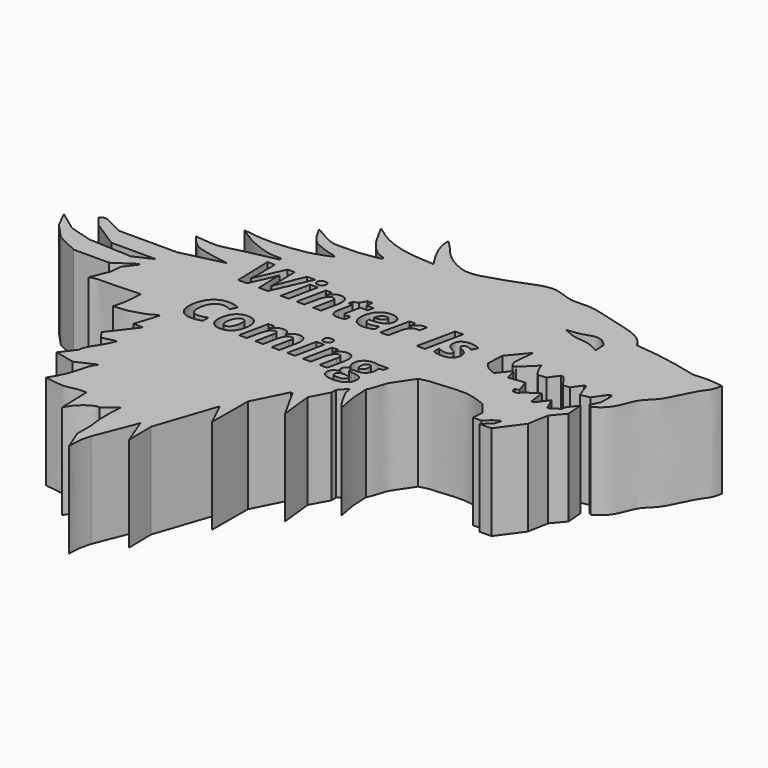
from build123d import *

# Parameters (mm, degrees)
F1_DEPTH     = 25
F2_R         = 94.3461279021
F3_DEPTH     = 25
F5_TEXT_SIZE = 14.0094855892
F6_DEPTH     = 25


# Not quite as in the source:
# - Text() gives the source's letters only with a copy of the font that has no kerning and outlines rounded to 1/6400 em; it was checked with that copy


with BuildPart() as f1:
    # F0 (on Top) → F1 (new body)
    with BuildSketch(Plane.XY):
        with BuildLine():
            add(Edge.make_bspline(
                [(8.3714025095, 46.0173152387), (11.1521832152, 46.754596787), (16.3296971789, 48.4982359497), (24.1106627679, 52.0612451404), (29.6085529308, 48.7695111991), (35.133174344, 49.9703703897), (43.252929809, 46.964556813), (51.3283334626, 45.612910231), (52.9993437231, 42.0622937381)],
                knots=[0, 0, 0, 0, 0.1755033114, 0.3449978942, 0.4876629093, 0.6241423562, 0.8019542951, 1, 1, 1, 1], degree=3))
            add(Edge.make_bspline(
                [(-6.1449650675, 54.0423952043), (-5.6293203869, 53.5672210533), (-4.3756327313, 52.4119294547), (-1.6804544816, 48.6615797252), (4.3028583968, 45.283770124), (7.1379722318, 45.7949318186), (8.3714025095, 46.0173152387)],
                knots=[0, 0, 0, 0, 0.18314369, 0.4452775175, 0.758665244, 1, 1, 1, 1], degree=3))
            add(Edge.make_bspline(
                [(-2.1649692208, 44.1456995904), (-2.6830426714, 44.902201383), (-3.8678058954, 46.6322176608), (-6.1266059516, 51.2050741718), (-6.1394772709, 53.1942802552), (-6.1449650675, 54.0423952043)],
                knots=[0, 0, 0, 0, 0.3083257044, 0.7050987754, 1, 1, 1, 1], degree=3))
            add(Edge.make_bspline(
                [(-20.5234307796, 49.826964736), (-19.2660471951, 48.8893211458), (-16.5760607157, 46.8833711627), (-10.5835555234, 44.6421995592), (-5.1143142903, 44.3196420651), (-2.1649692208, 44.1456995904)],
                knots=[0, 0, 0, 0, 0.2879457207, 0.6160173435, 1, 1, 1, 1], degree=3))
            add(Edge.make_bspline(
                [(-11.792646721, 39.9065613747), (-12.7415984122, 40.1991817878), (-14.864454764, 40.8537895075), (-17.9140349598, 44.889493557), (-18.9338887823, 46.9178849726), (-19.9665200349, 48.807741727), (-20.5234307796, 49.826964736)],
                knots=[0, 0, 0, 0, 0.242668036, 0.5428615453, 0.7534596047, 1, 1, 1, 1], degree=3))
            Line((-11.792646721, 39.9065613747), (-12.1578518301, 39.2757542431))
            Line((-12.1578518301, 39.2757542431), (-17.669133842, 38.4789407253))
            add(Edge.make_bspline(
                [(-30.1525183022, 41.5333881974), (-29.4462955799, 41.1485654195), (-27.8722301429, 40.2908526681), (-24.4388988209, 38.1832992198), (-20.9659487244, 38.4500592903), (-18.7606144745, 38.4693789125), (-17.669133842, 38.4789407253)],
                knots=[0, 0, 0, 0, 0.2218830142, 0.4945442459, 0.7498360323, 1, 1, 1, 1], degree=3))
            add(Edge.make_bspline(
                [(-20.9172498435, 34.4844385982), (-22.0652264332, 34.5773157469), (-24.8199894343, 35.715890512), (-27.6018886219, 36.794447921), (-29.4810709407, 40.069825786), (-30.1525183022, 41.5333881974)],
                knots=[0, 0, 0, 0, 0.3311370823, 0.6221258171, 1, 1, 1, 1], degree=3))
            add(Edge.make_bspline(
                [(-20.7182727754, 33.6885266006), (-20.3961660871, 33.7569314037), (-20.0173134256, 34.0869757025), (-20.4925501201, 34.2820213144), (-20.9172498435, 34.4844385982)],
                knots=[0, 0, 0, 0, 0.4600614089, 1, 1, 1, 1], degree=3))
            add(Edge.make_bspline(
                [(-41.9234707952, 31.6619388759), (-40.2252279309, 31.4070143382), (-36.7717771519, 30.8886141953), (-31.412260856, 31.079758672), (-24.6846617301, 32.0754797978), (-21.932813416, 33.1945985165), (-20.7182727754, 33.6885266006)],
                knots=[0, 0, 0, 0, 0.2445734873, 0.4973508312, 0.7781535267, 1, 1, 1, 1], degree=3))
            add(Edge.make_bspline(
                [(-28.4772720188, 26.5822634101), (-29.4158292377, 26.5659337389), (-31.6836604975, 26.5264764335), (-37.6292895418, 28.7001284099), (-40.5298935718, 30.7007517807), (-41.9234707952, 31.6619388759)],
                knots=[0, 0, 0, 0, 0.2683864124, 0.6485007876, 1, 1, 1, 1], degree=3))
            ThreePointArc((-28.4772720188, 26.5822634101), (-28.1204352447, 26.2336581945), (-28.4772720188, 25.885052979))
            add(Edge.make_bspline(
                [(-47.9933172464, 23.3067888767), (-45.9689231613, 23.0397900521), (-42.1158191567, 22.5316013316), (-37.515328371, 24.0476780795), (-31.8113888815, 25.2072498766), (-28.4772720188, 25.885052979)],
                knots=[0, 0, 0, 0, 0.3150353706, 0.5996184522, 1, 1, 1, 1], degree=3))
            add(Edge.make_bspline(
                [(-35.507440567, 17.9841239005), (-37.7337411291, 18.2148626084), (-41.7881476434, 19.1150723529), (-45.0286914617, 19.7872195383), (-47.2463314192, 22.1207634071), (-47.9933172464, 23.3067888767)],
                knots=[0, 0, 0, 0, 0.3933673205, 0.675332231, 1, 1, 1, 1], degree=3))
            add(Edge.make_bspline(
                [(-46.6502159834, 15.3476633132), (-44.9365327779, 15.7569410645), (-41.3990675416, 16.601791392), (-37.5116464679, 17.5138838493), (-35.507440567, 17.9841239005)],
                knots=[0, 0, 0, 0, 0.4844381756, 1, 1, 1, 1], degree=3))
            Line((-46.6502159834, 15.3476633132), (-62.0212741196, 15.3476633132))
            Line((-62.0212741196, 15.3476633132), (-66.7967498302, 17.8348906338))
            add(Edge.make_bspline(
                [(-68.9357668161, 17.4369327724), (-68.6066134375, 17.6698578481), (-67.9506292373, 18.1340644442), (-67.1804673623, 17.9343795713), (-66.7967498302, 17.8348906338)],
                knots=[0, 0, 0, 0, 0.5017702843, 1, 1, 1, 1], degree=3))
            Line((-68.9357668161, 17.4369327724), (-66.8741110966, 14.7528935398))
            Line((-66.8741110966, 14.7528935398), (-59.8598131947, 10.2239763364))
            Line((-59.8598131947, 10.2239763364), (-48.1540286598, 10.2239763364))
            Line((-48.1540286598, 10.2239763364), (-52.9180280864, 7.9854726791))
            Line((-52.9180280864, 7.9854726791), (-64.2597824335, 8.5326619446))
            Line((-64.2597824335, 8.5326619446), (-70.2788680792, 10.2737210691))
            Line((-70.2788680792, 10.2737210691), (-75.4522979259, 14.1040496528))
            Line((-75.4522979259, 14.1040496528), (-73.263540864, 9.7265308723))
            Line((-73.263540864, 9.7265308723), (-69.4829523563, 5.6474790908))
            Line((-69.4829523563, 5.6474790908), (-63.9623478055, 2.9811237473))
            Line((-63.9623478055, 2.9811237473), (-54.6376407146, 2.9811237473))
            Line((-54.6376407146, 2.9811237473), (-49.4906404484, 6.4263421627))
            Line((-49.4906404484, 6.4263421627), (-49.2154881358, 6.2145185657))
            Line((-49.2154881358, 6.2145185657), (-51.6280978918, 3.0806129798))
            Line((-51.6280978918, 3.0806129798), (-51.8768206239, 0.2700467885))
            Line((-51.8768206239, 0.2700467885), (-53.897228092, -4.7841728665))
            add(Edge.make_bspline(
                [(-40.8291891217, -3.9497618563), (-42.0186421901, -3.8093417167), (-45.3107909022, -4.0968469373), (-48.3842299956, -4.2614385352), (-52.4190030992, -3.9870282635), (-53.897228092, -4.7841728665)],
                knots=[0, 0, 0, 0, 0.3316033773, 0.6282267504, 1, 1, 1, 1], degree=3))
            add(Edge.make_bspline(
                [(-41.9053472579, -11.5949641913), (-41.6162947666, -10.5393210499), (-40.9622835051, -8.2946564661), (-40.9048251743, -5.3812860287), (-40.8291891217, -3.9497618563)],
                knots=[0, 0, 0, 0, 0.4692918634, 1, 1, 1, 1], degree=3))
            add(Edge.make_bspline(
                [(-31.7871761994, -8.8916057721), (-32.2743129695, -8.782544191), (-34.030595376, -10.1978115242), (-36.188481433, -10.5333033514), (-38.2784013347, -11.4723443654), (-41.0598919467, -11.5172522083), (-41.9053472579, -11.5949641913)],
                knots=[0, 0, 0, 0, 0.2398632365, 0.4733244812, 0.7104125663, 1, 1, 1, 1], degree=3))
            Line((-31.7871761994, -8.8916057721), (-33.7395146489, -15.1539025828))
            Line((-33.7395146489, -15.1539025828), (-31.2054082751, -15.1539025828))
            Line((-31.2054082751, -15.1539025828), (-36.57175228, -22.1599657089))
            Line((-36.57175228, -22.1599657089), (-35.0811034441, -24.0978132933))
            Line((-35.0811034441, -24.0978132933), (-31.5780714154, -23.2779551297))
            add(Edge.make_bspline(
                [(-35.3792309761, -31.252939254), (-35.2093878882, -30.5393633822), (-34.822538413, -28.9140605517), (-32.4597849698, -25.8039051405), (-31.8536027802, -24.0673027021), (-31.5780714154, -23.2779551297)],
                knots=[0, 0, 0, 0, 0.2991875934, 0.681455836, 1, 1, 1, 1], degree=3))
            Line((-35.3792309761, -31.252939254), (-38.1369404495, -34.905038774))
            Line((-38.1369404495, -34.905038774), (-32.9941920936, -36.0975600779))
            Line((-32.9941920936, -36.0975600779), (-27.9259737581, -33.7870493531))
            add(Edge.make_bspline(
                [(-32.8369960189, -45.0255796313), (-31.8515502928, -43.5405302157), (-30.2705672919, -40.7462703248), (-29.4369524253, -36.660524163), (-28.6514393679, -34.6910328201), (-27.9259737581, -33.7870493531)],
                knots=[0, 0, 0, 0, 0.3712531138, 0.7036510455, 1, 1, 1, 1], degree=3))
            add(Edge.make_bspline(
                [(-22.2036093473, -45.0255796313), (-22.772011898, -45.0397864605), (-23.7004218348, -44.9797600854), (-25.4254406404, -45.1837723147), (-27.7325988764, -45.919739897), (-30.3529637151, -45.3235164981), (-32.2593170359, -45.2133178015), (-32.8369960189, -45.0255796313)],
                knots=[0, 0, 0, 0, 0.168563403, 0.346643991, 0.5578300792, 0.7864867179, 1, 1, 1, 1], degree=3))
            Line((-22.2036093473, -45.0255796313), (-21.956436336, -53.3252209425))
            add(Edge.make_bspline(
                [(-15.8648324454, -48.5923998058), (-16.1901104984, -48.5404788164), (-16.9341453944, -48.3881727953), (-20.0429975744, -50.2948936774), (-21.2835316, -52.2014005669), (-21.956436336, -53.3252209425)],
                knots=[0, 0, 0, 0, 0.2088779675, 0.5927214975, 1, 1, 1, 1], degree=3))
            Line((-15.8648324454, -48.5923998058), (-12.4351317063, -45.8902679384))
            add(Edge.make_bspline(
                [(-12.2157726437, -55.672917515), (-12.4860550779, -54.5293685296), (-12.6693441086, -52.4229659715), (-12.7064015911, -47.8621878063), (-12.4871159035, -46.4728990449), (-12.4351317063, -45.8902679384)],
                knots=[0, 0, 0, 0, 0.3448325876, 0.7390589855, 1, 1, 1, 1], degree=3))
            Line((-12.2157726437, -55.672917515), (-12.2157726437, -60.5109594567))
            Line((-12.2157726437, -60.5109594567), (-10.078990832, -65.9852549434))
            add(Edge.make_bspline(
                [(-9.2842206359, -59.7107559443), (-9.4550305782, -60.5384345816), (-9.902582499, -61.8062985958), (-10.0438074046, -63.8134681556), (-10.1501073839, -64.8883362759), (-10.078990832, -65.9852549434)],
                knots=[0, 0, 0, 0, 0.3434410399, 0.6516969652, 1, 1, 1, 1], degree=3))
            Line((-9.2842206359, -59.7107559443), (-4.9888626672, -48.7853176892))
            Line((-4.9888626672, -48.7853176892), (-2.1685243119, -56.0555234551))
            Line((-2.1685243119, -56.0555234551), (-2.293872647, -48.6599691212))
            Line((-2.293872647, -48.6599691212), (3.0732932501, -32.7431671321))
            Line((3.0732932501, -32.7431671321), (6.1721643433, -39.175670594))
            Line((6.1721643433, -39.175670594), (6.2191165052, -27.43752487))
            Line((6.2191165052, -27.43752487), (10.6033291668, -18.757302314))
            Line((10.6033291668, -18.757302314), (11.119807139, -18.8512075692))
            Line((11.119807139, -18.8512075692), (15.5803030357, -26.9270520657))
            Line((15.5803030357, -26.9270520657), (14.641251415, -18.2877760381))
            Line((14.641251415, -18.2877760381), (17.1766914427, -13.5567625985))
            Line((17.1766914427, -13.5567625985), (17.1766914427, -12.0627405122))
            Line((17.1766914427, -12.0627405122), (19.1386900842, -9.8922895268))
            Line((19.1386900842, -9.8922895268), (19.4833967835, -11.8665257469))
            add(Edge.make_bspline(
                [(19.4833967835, -11.8665257469), (19.9582581906, -12.7343634222), (20.8940276903, -14.6410966661), (22.20068118, -16.664738753), (23.0558253825, -17.7265629172)],
                knots=[0, 0, 0, 0, 0.4722933866, 1, 1, 1, 1], degree=3))
            add(Edge.make_bspline(
                [(21.8564793468, -8.0677578226), (21.9043409964, -9.664840016), (21.9482815798, -12.5516169935), (22.6847221236, -16.0473406273), (23.0558253825, -17.7265629172)],
                knots=[0, 0, 0, 0, 0.4822099629, 1, 1, 1, 1], degree=3))
            add(Edge.make_bspline(
                [(27.2579398006, 2.3084669374), (26.1194505133, 0.492341682), (24.3268514422, -2.2289048112), (23.6689481263, -2.9581086655), (23.0922805979, -4.6614855998), (22.6014648499, -6.7147728959), (21.8564793468, -8.0677578226)],
                knots=[0, 0, 0, 0, 0.3601937688, 0.5069047837, 0.6994256048, 1, 1, 1, 1], degree=3))
            add(Edge.make_bspline(
                [(44.5988215506, 1.7908602022), (42.8253273849, 2.5411266674), (39.1136452825, 4.1113323467), (31.2287135334, 2.8018420649), (30.2677562277, 3.0778660852), (28.4262352341, 2.6071182116), (27.2579398006, 2.3084669374)],
                knots=[0, 0, 0, 0, 0.3130703353, 0.6552136357, 0.7812610683, 1, 1, 1, 1], degree=3))
            Line((44.5988215506, 1.7908602022), (47.0203794539, -1.2552264379))
            Line((47.0203794539, -1.2552264379), (46.8641519547, -4.0865577757))
            Line((46.8641519547, -4.0865577757), (49.0708984435, -4.0865577757))
            Line((49.0708984435, -4.0865577757), (50.6527237594, -2.56305933))
            Line((50.6527237594, -2.56305933), (52.4207316339, -1.5848465264))
            Line((52.4207316339, -1.5848465264), (51.9937686622, -3.292765934))
            Line((51.9937686622, -3.292765934), (49.7275851667, -5.4931365885))
            Line((49.7275851667, -5.4931365885), (52.7820065618, -5.4931365885))
            Line((52.7820065618, -5.4931365885), (57.3800653219, 0.7478338666))
            Line((57.3800653219, 0.7478338666), (58.3653636277, 6.2328204513))
            Line((58.3653636277, 6.2328204513), (61.1234270036, 9.5133176073))
            Line((61.1234270036, 9.5133176073), (60.7547722757, 13.8265006244))
            Line((60.7547722757, 13.8265006244), (58.8009096682, 11.2456092611))
            Line((58.8009096682, 11.2456092611), (58.6903169751, 10.2870920673))
            Line((58.6903169751, 10.2870920673), (56.1466068029, 8.6646042764))
            Line((56.1466068029, 8.6646042764), (54.635129869, 12.0191024616))
            Line((54.635129869, 12.0191024616), (52.3494780064, 8.9588118717))
            Line((52.3494780064, 8.9588118717), (51.7596304417, 8.9588118717))
            Line((51.7596304417, 8.9588118717), (51.1783212423, 13.1371170282))
            Line((51.1783212423, 13.1371170282), (47.7149188519, 10.900686495))
            add(Edge.make_bspline(
                [(47.7149188519, 10.900686495), (47.5838957556, 10.6244864745), (47.2974333019, 10.0206163338), (45.6467267018, 10.0257036878), (45.6102647492, 10.7669772696), (45.5935673907, 11.1064355238)],
                knots=[0, 0, 0, 0, 0.3136178749, 0.6856786973, 1, 1, 1, 1], degree=3))
            Line((45.5935673907, 11.1064355238), (46.6129109263, 11.4333555102))
            Line((46.6129109263, 11.4333555102), (45.5335724738, 14.7987559755))
            Line((45.5335724738, 14.7987559755), (41.3075014949, 14.2341526225))
            Line((41.3075014949, 14.2341526225), (40.6942255795, 16.9787928462))
            Line((40.6942255795, 16.9787928462), (40.2023345232, 16.9787928462))
            Line((40.2023345232, 16.9787928462), (37.8335155547, 14.0522215515))
            add(Edge.make_bspline(
                [(34.1536141932, 16.5792405605), (34.7159098959, 15.9995110541), (35.5539627286, 14.80137631), (37.1673543775, 14.3088527408), (37.8335155547, 14.0522215515)],
                knots=[0, 0, 0, 0, 0.4981977471, 1, 1, 1, 1], degree=3))
            Line((34.1536141932, 16.5792405605), (34.3964099884, 21.1116671562))
            Line((34.3964099884, 21.1116671562), (38.5461710393, 26.1463858187))
            Line((38.5461710393, 26.1463858187), (38.0535237491, 20.5301064998))
            add(Edge.make_bspline(
                [(38.0535237491, 20.5301064998), (38.1200252746, 20.2667031932), (38.2566733374, 19.7254591944), (38.8369682468, 18.760294285), (39.3575997521, 18.9603562109), (39.5971573889, 19.0524104983)],
                knots=[0, 0, 0, 0, 0.3385446369, 0.695645227, 1, 1, 1, 1], degree=3))
            Line((39.5971573889, 19.0524104983), (43.4069782495, 22.7643214166))
            add(Edge.make_bspline(
                [(45.5089472234, 19.0205313265), (45.0502235886, 19.2706052938), (44.3409213434, 20.4331289609), (43.6673983857, 21.7331408927), (43.4069782495, 22.7643214166)],
                knots=[0, 0, 0, 0, 0.4456569875, 1, 1, 1, 1], degree=3))
            Line((45.5089472234, 19.0205313265), (47.5452281535, 19.2507654428))
            Line((47.5452281535, 19.2507654428), (49.3639968336, 21.7646621168))
            Line((49.3639968336, 21.7646621168), (49.9640069902, 21.7646621168))
            Line((49.9640069902, 21.7646621168), (52.3847304285, 18.6408720911))
            Line((52.3847304285, 18.6408720911), (54.0192387998, 18.8273470849))
            Line((54.0192387998, 18.8273470849), (55.7778850198, 21.3104300201))
            Line((55.7778850198, 21.3104300201), (56.3235357404, 21.320130676))
            Line((56.3235357404, 21.320130676), (57.7169582248, 17.5116695464))
            Line((57.7169582248, 17.5116695464), (60.085773468, 17.9765298963))
            Line((60.085773468, 17.9765298963), (62.4545887113, 21.3211290538))
            Line((62.4545887113, 21.3211290538), (63.1977468729, 21.1819000542))
            Line((63.1977468729, 21.1819000542), (63.1977468729, 17.6983531564))
            Line((63.1977468729, 17.6983531564), (61.9901157916, 15.2364429086))
            Line((61.9901157916, 15.2364429086), (62.7864152193, 14.6962208673))
            add(Edge.make_bspline(
                [(78.0018940568, 38.8766825199), (77.8942045693, 37.8249602858), (77.2752538197, 35.8416326235), (75.2928965724, 33.857636495), (72.2717646913, 26.0114297278), (68.2536757327, 23.5239123526), (66.8766638895, 17.530828089), (64.1988176388, 15.4915865184), (62.7864152193, 14.6962208673)],
                knots=[0, 0, 0, 0, 0.1323192519, 0.2623037717, 0.4807629009, 0.6483524821, 0.8307680207, 1, 1, 1, 1], degree=3))
            add(Edge.make_bspline(
                [(70.1987296343, 39.0611998737), (71.4230337563, 39.1671903489), (73.9332266725, 39.3845028086), (76.6236692988, 39.0487021097), (78.0018940568, 38.8766825199)],
                knots=[0, 0, 0, 0, 0.4877330798, 1, 1, 1, 1], degree=3))
            add(Edge.make_bspline(
                [(52.9993437231, 42.0622937381), (55.9223519783, 41.8244427562), (62.0327163544, 41.046729132), (67.3881612896, 39.8143175247), (70.1987296343, 39.0611998737)],
                knots=[0, 0, 0, 0, 0.5076004824, 1, 1, 1, 1], degree=3))
        make_face()
        with BuildLine():
            add(Edge.make_bspline(
                [(37.4237261713, 38.3135154843), (38.5139452229, 37.7823419639), (40.7086892192, 36.7202854022), (44.4869246995, 36.8517157254), (46.7188540611, 35.6130370736), (47.8210225701, 34.9595472217)],
                knots=[0, 0, 0, 0, 0.3300229577, 0.6622621188, 1, 1, 1, 1], degree=3))
            add(Edge.make_bspline(
                [(37.4237261713, 38.3135154843), (38.9198290263, 38.4614281476), (40.7559340918, 38.5719885086), (43.6999611933, 39.9000659499), (46.1302772151, 39.5946865513), (47.3397361352, 38.2043084802), (47.709222883, 37.8290526569)],
                knots=[0, 0, 0, 0, 0.282952661, 0.5447082368, 0.7761041189, 1, 1, 1, 1], degree=3))
            Line((47.709222883, 37.8290526569), (47.8210225701, 34.9595472217))
        make_face(mode=Mode.SUBTRACT)
    extrude(amount=F1_DEPTH)

    # F5 (on face) → F6 (cut)
    with BuildSketch(Plane.XY.offset(25)):
        with Locations((-30.6766790897, 13.5297201468)):
            Text('Winter Is', F5_TEXT_SIZE, font='Open Sans', font_style=FontStyle.BOLDITALIC, text_align=(TextAlign.LEFT, TextAlign.BOTTOM))
        with Locations((-30.6766790897, -5.5231802545)):
            Text('Coming', F5_TEXT_SIZE, font='Open Sans', font_style=FontStyle.BOLDITALIC, text_align=(TextAlign.LEFT, TextAlign.BOTTOM))
    extrude(amount=-F6_DEPTH, mode=Mode.SUBTRACT)


with BuildPart() as f3:
    # F2 (on Top) → F3 (new body)
    with BuildSketch(Plane.XY):
        Circle(F2_R)
        with BuildLine():
            add(Edge.make_bspline(
                [(14.7567046806, 81.5834701061), (14.7567046806, 94.5155938661), (-7.3783523403, 88.0495319861), (-29.5134093612, 81.5834701061), (-7.3783523403, 75.1174082262), (14.7567046806, 68.6513463462), (14.7567046806, 81.5834701061)],
                knots=[0, 0, 0, 2.0943951024, 2.0943951024, 4.1887902048, 4.1887902048, 6.2831853072, 6.2831853072, 6.2831853072], degree=2, weights=[1, 0.5, 1, 0.5, 1, 0.5, 1]))
        make_face(mode=Mode.SUBTRACT)
    extrude(amount=F3_DEPTH)


solid = f1.part
